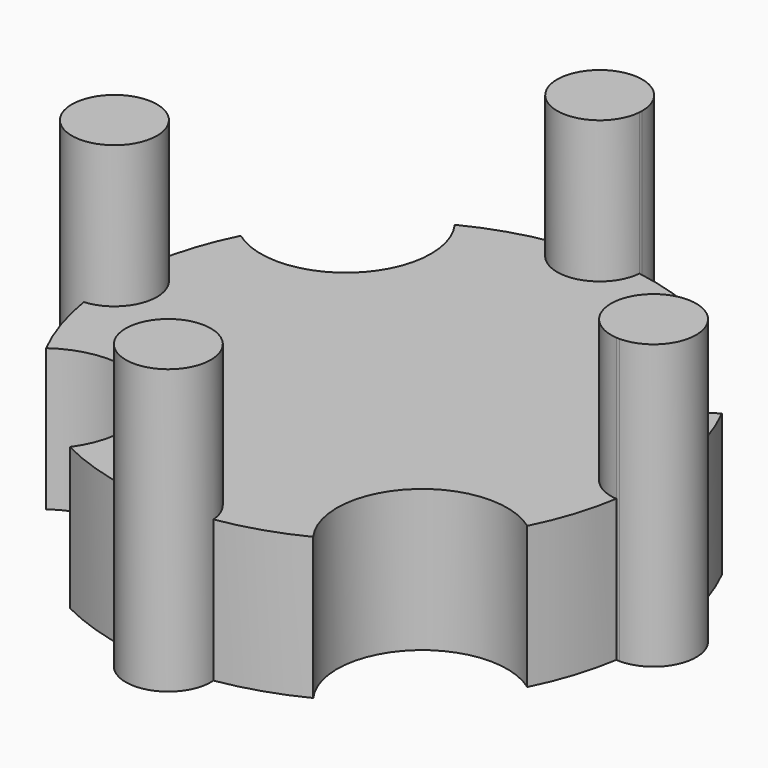
from build123d import *

# Parameters (mm, degrees)
F1_DEPTH        = 25
F2_DEPTH        = 50
F2_COPIES_COUNT = 4
F4_DEPTH        = 25.001
F4_COPIES_COUNT = 4


# Not quite as in the source:
# - a pattern or mirror of a feature is missing from the dataset's text; its kind, count and spacing are read off the source's solid


with BuildPart() as f1:
    # F0 (on Top) → F1 (new body)
    with BuildSketch(Plane.XY):
        with BuildLine():
            ThreePointArc((-7.4765908914, 46.9078947368), (-30.8310876605, -36.1343885194), (47.5, 0))
            ThreePointArc((47.5, 0), (36.1343885194, 30.8310876605), (7.4765908914, 46.9078947368))
            ThreePointArc((7.4765908914, 46.9078947368), (0, 40), (-7.4765908914, 46.9078947368))
        make_face()
        with BuildLine():
            ThreePointArc((-7.4765908914, 46.9078947368), (0, 40), (7.4765908914, 46.9078947368))
            ThreePointArc((7.4765908914, 46.9078947368), (0, 47.5), (-7.4765908914, 46.9078947368))
        make_face()
    extrude(amount=F1_DEPTH)

    # F0 (on Top) → F2 (join)
    with BuildSketch(Plane.XY):
        with BuildLine():
            ThreePointArc((-7.4765908914, 46.9078947368), (0, 40), (7.4765908914, 46.9078947368))
            ThreePointArc((7.4765908914, 46.9078947368), (0, 47.5), (-7.4765908914, 46.9078947368))
        make_face()
        with BuildLine():
            ThreePointArc((-7.4765908914, 46.9078947368), (0, 47.5), (7.4765908914, 46.9078947368))
            ThreePointArc((7.4765908914, 46.9078947368), (7.4941454378, 47.2037160867), (7.5, 47.5))
            ThreePointArc((7.5, 47.5), (-0.2962839133, 54.9941454378), (-7.4765908914, 46.9078947368))
        make_face()
    f2 = extrude(amount=F2_DEPTH)

    # F2_copies: F2 ×4 about axis
    f2_copies_axis = Axis((0, 0, 0), (0, 0, 1))
    for i in range(1, F2_COPIES_COUNT):
        add(f2.rotate(f2_copies_axis, i * 360 / F2_COPIES_COUNT))

    # F3 (on face) → F4 (cut, through all)
    with BuildSketch(Plane.XY.offset(25)):
        with BuildLine():
            ThreePointArc((42.3863974889, 21.4392935498), (33.5875721064, 33.5875721064), (21.4392935498, 42.3863974889))
            ThreePointArc((21.4392935498, 42.3863974889), (22.9809703886, 22.9809703886), (42.3863974889, 21.4392935498))
        make_face()
    f4 = extrude(amount=-F4_DEPTH, mode=Mode.SUBTRACT)

    # F4_copies: F4 ×4 about axis
    f4_copies_axis = Axis((0, 0, 0), (0, 0, 1))
    for i in range(1, F4_COPIES_COUNT):
        add(f4.rotate(f4_copies_axis, i * 360 / F4_COPIES_COUNT), mode=Mode.SUBTRACT)


solid = f1.part
